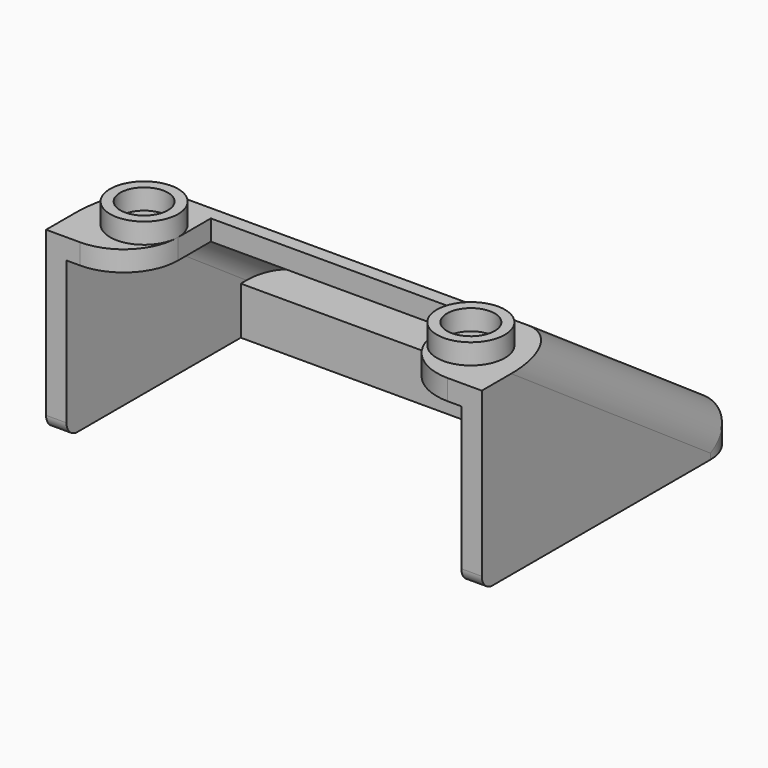
from build123d import *

# Parameters (mm, degrees)
F1_DEPTH     = 16
F2_R         = 3
F3_R         = 1.5
F4_DEPTH     = 2
F5_T         = 1.5
F5_T3_DEPTH  = 5
F5_T5_DEPTH  = 6.5
F5_T7_DEPTH  = 32
F5_T9_DEPTH  = 29
F5_T12_ANGLE = 90.000000001
F5_T14_ANGLE = 90.000000001
F7_DEPTH     = 13.001
F6_R         = 2.5
F6_R_2       = 1.75
F8_DEPTH     = 1.5
F9_R         = 1


# Not quite as in the source:
# - a shell that OpenCascade refuses in one call is made with other operations: the cavity is built on its own and cut out


with BuildPart() as f1:
    # F0 (on Right) → F1 (new body, symmetric)
    with BuildSketch(Plane.YZ):
        Polygon((12, -4.5), (-4, 6.5), (-12, 6.5), (-12, -6.5), (12, -6.5), align=None)
    extrude(amount=F1_DEPTH, both=True)

    # F2
    f2_edges = [f1.edges().sort_by_distance(p)[0] for p in [
        (16, 12, -5.5),
        (-16, 12, -5.5),
        (16, 4, 1),
        (-16, 4, 1),
    ]]
    fillet(f2_edges, radius=F2_R)

    # F3 (on face) → F4 (cut)
    with BuildSketch(Plane(origin=(0, 0, -6.5), x_dir=(1, 0, 0), z_dir=(0, 0, -1))):
        with BuildLine():
            ThreePointArc((13, -10.5), (14.0606601718, -10.0606601718), (14.5, -9))
            Line((14.5, -9), (14.5, -5.5))
            Line((14.5, -5.5), (-14.5, -5.5))
            Line((-14.5, -5.5), (-14.5, -9))
            ThreePointArc((-14.5, -9), (-14.0606601718, -10.0606601718), (-13, -10.5))
            Line((-13, -10.5), (13, -10.5))
        make_face()
        with Locations((-8, -8)):
            Circle(F3_R, mode=Mode.SUBTRACT)
        with Locations((0, -8)):
            Circle(F3_R, mode=Mode.SUBTRACT)
        with Locations((8, -8)):
            Circle(F3_R, mode=Mode.SUBTRACT)
    extrude(amount=-F4_DEPTH, mode=Mode.SUBTRACT)

    # F5: shell of thickness 1.5, made by hand


with BuildPart() as f5_core1:
    # F5_t2: copy of F1
    add(f1.part)

    # the walls: a layer under each face that stays
    f5_faces = [f5_core1.faces().sort_by_distance(p)[0] for p in [
        (0, 4, 1),
        (0, -8, 6.5),
        (-15.1213203436, 1.7042929957, 1.5119940115),
        (15.1213203436, 1.7042929957, 1.5119940115),
        (0, 12, -5.5),
        (-16, -1.5, 0),
        (16, -1.5, 0),
        (-15.1213203436, 11.1213203436, -5.5),
        (15.1213203436, 11.1213203436, -5.5),
        (14.0606601718, 10.0606601718, -5.5),
        (14.5, 7.25, -5.5),
        (0, 5.5, -5.5),
        (-14.5, 7.25, -5.5),
        (-14.0606601718, 10.0606601718, -5.5),
        (0, 10.5, -5.5),
        (-9.6666666667, 9.6666666667, -4.5),
        (-8, 8, -6.5),
        (0, 8, -6.5),
        (8, 8, -6.5),
    ]]
    thicken(f5_faces, amount=-F5_T, mode=Mode.SUBTRACT)

    # F5_s4 → F5_t3 (cut)
    with BuildSketch(Plane.XY.offset(-8)):
        Polygon((14.485, 5.515), (16, 5.5), (16, 4), (14.5, 4), align=None)
        Polygon((-14.485, 5.515), (-14.5, 4), (-16, 4), (-16, 5.5), align=None)
    extrude(amount=F5_T3_DEPTH, mode=Mode.SUBTRACT)

    # F5_s6 → F5_t5 (cut)
    with BuildSketch(Plane.XZ.offset(-10.5)):
        Polygon((14.485, -4.515), (16, -4.5), (16, -3), (14.5, -3), align=None)
        Polygon((-14.485, -4.515), (-16, -4.5), (-16, -3), (-14.5, -3), align=None)
    extrude(amount=F5_T5_DEPTH, mode=Mode.SUBTRACT)

    # F5_s8 → F5_t7 (cut)
    with BuildSketch(Plane.YZ.offset(-16)):
        Polygon((5.515, -4.515), (4, -4.5), (4, -3), (5.5, -3), align=None)
    extrude(amount=F5_T7_DEPTH, mode=Mode.SUBTRACT)

    # F5_s10 → F5_t9 (cut)
    with BuildSketch(Plane.YZ.offset(-14.5)):
        Polygon((10.485, -4.515), (12, -4.5), (12, -3), (10.5, -3), align=None)
    extrude(amount=F5_T9_DEPTH, mode=Mode.SUBTRACT)

    # F5_s11 → F5_t12 (revolve, cut)
    with BuildSketch(Plane.YZ.offset(13)):
        Polygon((10.485, -4.515), (12, -4.5), (12, -3), (10.5, -3), align=None)
    revolve(axis=Axis((13, 9, -4.5), (0, 0, -1)), revolution_arc=F5_T12_ANGLE, mode=Mode.SUBTRACT)

    # F5_s13 → F5_t14 (revolve, cut)
    with BuildSketch(Plane.XZ.offset(-9)):
        Polygon((-14.485, -4.515), (-16, -4.5), (-16, -3), (-14.5, -3), align=None)
    revolve(axis=Axis((-13, 9, -4.5), (0, 0, -1)), revolution_arc=F5_T14_ANGLE, mode=Mode.SUBTRACT)

    # F5_s15 → F5_t16 (revolve, cut)
    with BuildSketch(Plane.XZ.offset(-8)):
        Polygon((-6.485, -4.515), (-6.5, -3), (-8, -3), (-8, -4.5), align=None)
    revolve(axis=Axis((-8, 8, -4.5), (0, 0, -1)), mode=Mode.SUBTRACT)

    # F5_s17 → F5_t18 (revolve, cut)
    with BuildSketch(Plane.XZ.offset(-8)):
        Polygon((1.515, -4.515), (1.5, -3), (0, -3), (0, -4.5), align=None)
    revolve(axis=Axis((0, 8, -4.5), (0, 0, -1)), mode=Mode.SUBTRACT)

    # F5_s19 → F5_t20 (revolve, cut)
    with BuildSketch(Plane.XZ.offset(-8)):
        Polygon((9.515, -4.515), (9.5, -3), (8, -3), (8, -4.5), align=None)
    revolve(axis=Axis((8, 8, -4.5), (0, 0, -1)), mode=Mode.SUBTRACT)


with BuildPart() as f1_1:
    add(f1.part)

    # what is left inside the walls is the cavity
    f5_cavity = [f5_core1.part.solids().sort_by_distance(p)[0] for p in [
        (-4.833333, -4, -6.485),
    ]]
    add(f5_cavity, mode=Mode.SUBTRACT)

    # F6 (on face) → F7 (cut, through all)
    with BuildSketch(Plane.XY.offset(6.5)):
        with BuildLine():
            Line((9.5, -5), (-9.5, -5))
            Line((-9.5, -5), (-9.5, -8))
            ThreePointArc((-9.5, -8), (-10.6715728753, -10.8284271247), (-13.5, -12))
            Line((-13.5, -12), (13.5, -12))
            ThreePointArc((13.5, -12), (10.6715728753, -10.8284271247), (9.5, -8))
            Line((9.5, -8), (9.5, -5))
        make_face()
    extrude(amount=-F7_DEPTH, mode=Mode.SUBTRACT)

    # F6 (on face) → F8 (join)
    with BuildSketch(Plane.XY.offset(6.5)):
        with Locations((-12, -8)):
            Circle(F6_R)
        with Locations((-12, -8)):
            Circle(F6_R_2, mode=Mode.SUBTRACT)
        with BuildLine():
            ThreePointArc((14.5, -8), (12, -5.5), (9.5, -8))
            ThreePointArc((9.5, -8), (12, -10.5), (14.5, -8))
        make_face()
        with Locations((12, -8)):
            Circle(F6_R_2, mode=Mode.SUBTRACT)
    extrude(amount=F8_DEPTH)

    # F9
    f9_edges = [f1_1.edges().sort_by_distance(p)[0] for p in [
        (15.25, -12, -6.5),
        (-15.25, -12, -6.5),
    ]]
    fillet(f9_edges, radius=F9_R)


solid = f1_1.part
